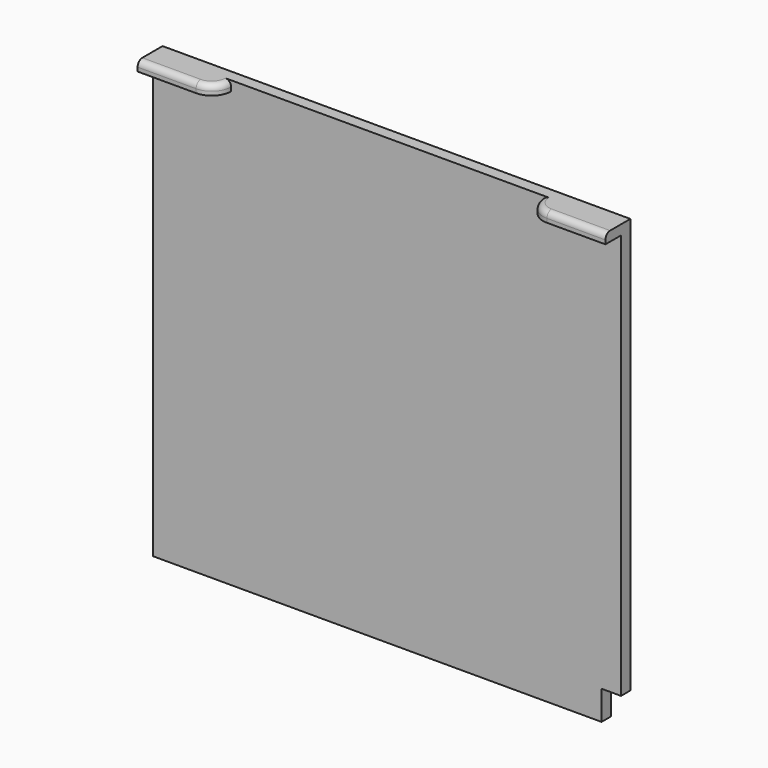
from build123d import *

# Parameters (mm, degrees)
F0_W     = 120
F0_H     = 114
F1_DEPTH = 3
F2_W     = 20
F2_H     = 2.5
F3_DEPTH = 5
F4_R     = 4.99999
F5_R     = 1.5
F6_W     = 5
F6_H     = 7.5
F7_DEPTH = 25


# Not quite as in the source:
# - a fillet or chamfer is up to 0.001 mm smaller than in the source, because OpenCascade refuses the exact size


with BuildPart() as f1:
    # F0 (on Front) → F1 (new body)
    with BuildSketch(Plane.XZ):
        with Locations((60, 57)):
            Rectangle(F0_W, F0_H)
    extrude(amount=F1_DEPTH)

    # F2 (on face) → F3 (join)
    with BuildSketch(Plane.XZ.offset(3)):
        with Locations((10, 112.75)):
            Rectangle(F2_W, F2_H)
        with Locations((110, 112.75)):
            Rectangle(F2_W, F2_H)
    extrude(amount=F3_DEPTH)

    # F4 (radius 5 in the source; OpenCascade refuses exactly that, so slightly less here)
    f4_edges = [f1.edges().sort_by_distance(p)[0] for p in [
        (20, -8, 112.75),
        (100, -8, 112.75),
    ]]
    fillet(f4_edges, radius=F4_R)

    # F5
    f5_edges = [f1.edges().sort_by_distance(p)[0] for p in [
        (7.500005, -8, 114),
        (112.499995, -8, 114),
    ]]
    fillet(f5_edges, radius=F5_R)

    # F6 (on face) → F7 (cut)
    with BuildSketch(Plane(origin=(0, 0, 0), x_dir=(-1, 0, 0), z_dir=(0, 1, 0))):
        with Locations((-117.5, 3.75)):
            Rectangle(F6_W, F6_H)
    extrude(amount=-F7_DEPTH, mode=Mode.SUBTRACT)


solid = f1.part
